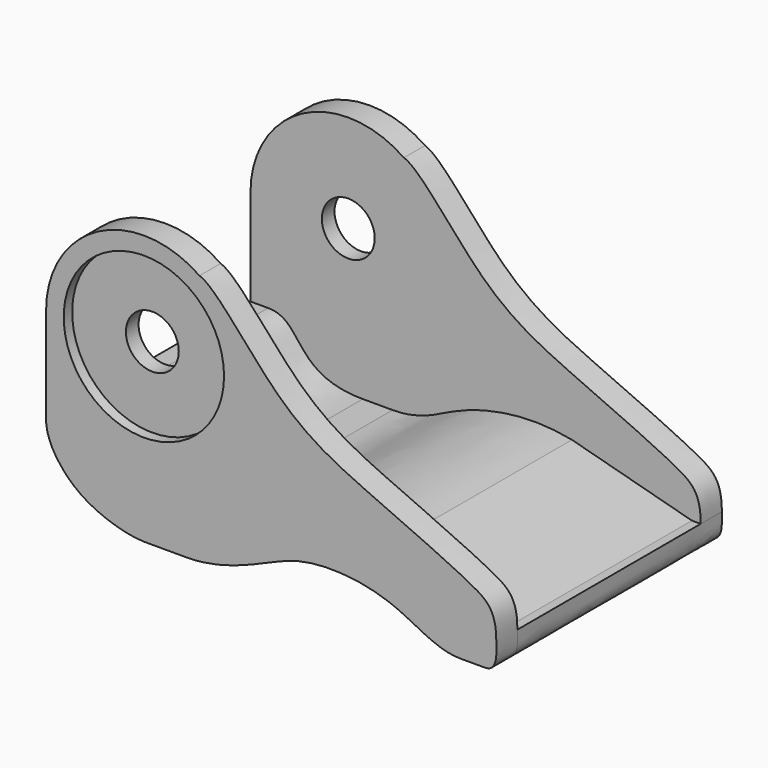
from build123d import *

# Parameters (mm, degrees)
F0_R     = 9.1
F0_R_2   = 3
F1_DEPTH = 3
F2_DEPTH = 32
F3_R     = 9.1
F3_R_2   = 3
F4_DEPTH = 3
F5_DEPTH = 1.2
F6_DEPTH = 1.2


# Not quite as in the source:
# - the dataset's text gives a spline's control points without its knots; the knots are read off the source's solid


with BuildPart() as f1:
    # F0 (on Front) → F1 (new body)
    with BuildSketch(Plane.XZ):
        with BuildLine():
            ThreePointArc((17.4131177763, 28.6298709707), (5.94566238, 29.330707182), (0, 19.5000000088))
            ThreePointArc((0, 19.5000000088), (11.0999999956, 8.4), (22.2, 19.5))
            ThreePointArc((22.2, 19.5), (20.93070718, 24.6543376239), (17.4131177763, 28.6298709707))
        make_face()
        with Locations((11.1, 19.5)):
            Circle(F0_R, mode=Mode.SUBTRACT)
        with BuildLine():
            Line((0, 19.5000000088), (0, 8.6))
            Line((0, 8.6), (2, 8.6))
            add(Edge.make_bspline(
                [(2, 8.6), (6.1005279422, 8.6), (4.7618634999, 3), (12.7434981987, 3)],
                knots=[0, 0, 0, 0, 12.1153932477, 12.1153932477, 12.1153932477, 12.1153932477], degree=3))
            Line((12.7434981987, 3), (16.1323161151, 3))
            add(Edge.make_bspline(
                [(36.4871002909, 6.6475654837), (33.250513749, 7.2772264404), (28.4821757642, 7.0333812875), (22.7707461668, 5.2870830071), (19.2182583484, 3), (16.1323161151, 3)],
                knots=[0, 0, 0, 0, 0.3619231415, 0.6598619876, 1, 1, 1, 1], degree=3))
            Line((36.4871002909, 6.6475654837), (50.1, 3))
            Line((50.1, 3), (51.1, 3))
            add(Edge.make_bspline(
                [(17.4131177763, 28.6298709707), (19.3173309809, 28.0148434267), (26.5141621262, 17.8054561903), (36.3055294732, 13.2861047363), (48.6152121195, 7.9013395134), (51.1, 6.0645417062), (51.1, 3)],
                knots=[0, 0, 0, 0, 0.2751149516, 0.5468245458, 0.818510602, 1, 1, 1, 1], degree=3))
            ThreePointArc((17.4131177763, 28.6298709707), (20.93070718, 24.6543376239), (22.2, 19.5))
            ThreePointArc((22.2, 19.5), (11.0999999956, 8.4), (0, 19.5000000088))
        make_face()
        with Locations((11.1, 19.5)):
            Circle(F0_R)
        with Locations((11.1, 19.5)):
            Circle(F0_R_2, mode=Mode.SUBTRACT)
        with BuildLine():
            add(Edge.make_bspline(
                [(36.4871002909, 6.6475654837), (33.250513749, 7.2772264404), (28.4821757642, 7.0333812875), (22.7707461668, 5.2870830071), (19.2182583484, 3), (16.1323161151, 3)],
                knots=[0, 0, 0, 0, 0.3619231415, 0.6598619876, 1, 1, 1, 1], degree=3))
            Line((16.1323161151, 3), (26.4085768866, 3))
            add(Edge.make_bspline(
                [(38.9945048839, 3), (37.6672047291, 3.494469873), (34.5451444696, 4.2269106386), (29.9007307702, 4.2671179583), (27.2729407986, 3.3486511872), (26.4085768866, 3)],
                knots=[0.2580240809, 0.2580240809, 0.2580240809, 0.2580240809, 0.396530844, 0.588257037, 0.6815213918, 0.6815213918, 0.6815213918, 0.6815213918], degree=3))
            Line((38.9945048839, 3), (50.1, 3))
            Line((50.1, 3), (36.4871002909, 6.6475654837))
        make_face()
        with BuildLine():
            Line((12.7434981987, 3), (3.1549932572, 3))
            add(Edge.make_bspline(
                [(11.1625680027, 0), (9.6983325574, 0), (6.2580804616, 0.8511709187), (3.8354236598, 2.4325332537), (3.1549932572, 3)],
                knots=[0, 0, 0, 0, 0.3599781606, 0.5310380634, 0.5310380634, 0.5310380634, 0.5310380634], degree=3))
            Line((11.1625680027, 0), (15.8881638199, 0))
            add(Edge.make_bspline(
                [(26.4085768866, 3), (25.5236936564, 2.6430721083), (22.55665667, 1.2844222732), (18.8493595825, 0), (15.8881638199, 0)],
                knots=[0.6815213918, 0.6815213918, 0.6815213918, 0.6815213918, 0.776999769, 1, 1, 1, 1], degree=3))
            Line((26.4085768866, 3), (16.1323161151, 3))
            Line((16.1323161151, 3), (12.7434981987, 3))
        make_face()
        with BuildLine():
            add(Edge.make_bspline(
                [(51.1, 3), (51.1, 1.8280865625), (51.3270497322, 0), (49.7638843954, 0)],
                knots=[0, 0, 0, 0, 3.2840835722, 3.2840835722, 3.2840835722, 3.2840835722], degree=3))
            Line((51.1, 3), (50.1, 3))
            Line((50.1, 3), (38.9945048839, 3))
            add(Edge.make_bspline(
                [(46.9955906657, 0), (44.6339409881, 0), (41.9557123636, 1.7760040782), (39.4711509433, 2.8224311844), (38.9945048839, 3)],
                knots=[0, 0, 0, 0, 0.2082849902, 0.2580240809, 0.2580240809, 0.2580240809, 0.2580240809], degree=3))
            Line((46.9955906657, 0), (49.7638843954, 0))
        make_face()
        with BuildLine():
            add(Edge.make_bspline(
                [(3.1549932572, 3), (2.7317734101, 3.3529577584), (2.3472268202, 3.728382037), (2, 4.1220149827)],
                knots=[0.5310380634, 0.5310380634, 0.5310380634, 0.5310380634, 0.6374353462, 0.6374353462, 0.6374353462, 0.6374353462], degree=3))
            Line((3.1549932572, 3), (12.7434981987, 3))
            add(Edge.make_bspline(
                [(2, 8.6), (6.1005279422, 8.6), (4.7618634999, 3), (12.7434981987, 3)],
                knots=[0, 0, 0, 0, 12.1153932477, 12.1153932477, 12.1153932477, 12.1153932477], degree=3))
            Line((2, 8.6), (2, 4.1220149827))
        make_face()
        with BuildLine():
            Line((2, 8.6), (0, 8.6))
            add(Edge.make_bspline(
                [(2, 4.1220149827), (1.7860800359, 4.3645248947), (0.6812014398, 5.7441151101), (0, 7.3046851351), (0, 8.6)],
                knots=[0.6374353462, 0.6374353462, 0.6374353462, 0.6374353462, 0.7029847265, 1, 1, 1, 1], degree=3))
            Line((2, 4.1220149827), (2, 8.6))
        make_face()
    extrude(amount=-F1_DEPTH)

    # F0 (on Front) → F2 (join)
    with BuildSketch(Plane.XZ):
        with BuildLine():
            Line((12.7434981987, 3), (3.1549932572, 3))
            add(Edge.make_bspline(
                [(11.1625680027, 0), (9.6983325574, 0), (6.2580804616, 0.8511709187), (3.8354236598, 2.4325332537), (3.1549932572, 3)],
                knots=[0, 0, 0, 0, 0.3599781606, 0.5310380634, 0.5310380634, 0.5310380634, 0.5310380634], degree=3))
            Line((11.1625680027, 0), (15.8881638199, 0))
            add(Edge.make_bspline(
                [(26.4085768866, 3), (25.5236936564, 2.6430721083), (22.55665667, 1.2844222732), (18.8493595825, 0), (15.8881638199, 0)],
                knots=[0.6815213918, 0.6815213918, 0.6815213918, 0.6815213918, 0.776999769, 1, 1, 1, 1], degree=3))
            Line((26.4085768866, 3), (16.1323161151, 3))
            Line((16.1323161151, 3), (12.7434981987, 3))
        make_face()
        with BuildLine():
            Line((2, 8.6), (0, 8.6))
            add(Edge.make_bspline(
                [(2, 4.1220149827), (1.7860800359, 4.3645248947), (0.6812014398, 5.7441151101), (0, 7.3046851351), (0, 8.6)],
                knots=[0.6374353462, 0.6374353462, 0.6374353462, 0.6374353462, 0.7029847265, 1, 1, 1, 1], degree=3))
            Line((2, 4.1220149827), (2, 8.6))
        make_face()
        with BuildLine():
            add(Edge.make_bspline(
                [(36.4871002909, 6.6475654837), (33.250513749, 7.2772264404), (28.4821757642, 7.0333812875), (22.7707461668, 5.2870830071), (19.2182583484, 3), (16.1323161151, 3)],
                knots=[0, 0, 0, 0, 0.3619231415, 0.6598619876, 1, 1, 1, 1], degree=3))
            Line((16.1323161151, 3), (26.4085768866, 3))
            add(Edge.make_bspline(
                [(38.9945048839, 3), (37.6672047291, 3.494469873), (34.5451444696, 4.2269106386), (29.9007307702, 4.2671179583), (27.2729407986, 3.3486511872), (26.4085768866, 3)],
                knots=[0.2580240809, 0.2580240809, 0.2580240809, 0.2580240809, 0.396530844, 0.588257037, 0.6815213918, 0.6815213918, 0.6815213918, 0.6815213918], degree=3))
            Line((38.9945048839, 3), (50.1, 3))
            Line((50.1, 3), (36.4871002909, 6.6475654837))
        make_face()
        with BuildLine():
            add(Edge.make_bspline(
                [(51.1, 3), (51.1, 1.8280865625), (51.3270497322, 0), (49.7638843954, 0)],
                knots=[0, 0, 0, 0, 3.2840835722, 3.2840835722, 3.2840835722, 3.2840835722], degree=3))
            Line((51.1, 3), (50.1, 3))
            Line((50.1, 3), (38.9945048839, 3))
            add(Edge.make_bspline(
                [(46.9955906657, 0), (44.6339409881, 0), (41.9557123636, 1.7760040782), (39.4711509433, 2.8224311844), (38.9945048839, 3)],
                knots=[0, 0, 0, 0, 0.2082849902, 0.2580240809, 0.2580240809, 0.2580240809, 0.2580240809], degree=3))
            Line((46.9955906657, 0), (49.7638843954, 0))
        make_face()
        with BuildLine():
            add(Edge.make_bspline(
                [(3.1549932572, 3), (2.7317734101, 3.3529577584), (2.3472268202, 3.728382037), (2, 4.1220149827)],
                knots=[0.5310380634, 0.5310380634, 0.5310380634, 0.5310380634, 0.6374353462, 0.6374353462, 0.6374353462, 0.6374353462], degree=3))
            Line((3.1549932572, 3), (12.7434981987, 3))
            add(Edge.make_bspline(
                [(2, 8.6), (6.1005279422, 8.6), (4.7618634999, 3), (12.7434981987, 3)],
                knots=[0, 0, 0, 0, 12.1153932477, 12.1153932477, 12.1153932477, 12.1153932477], degree=3))
            Line((2, 8.6), (2, 4.1220149827))
        make_face()
    extrude(amount=-F2_DEPTH)

    # F3 (on face) → F4 (join)
    with BuildSketch(Plane(origin=(0, 32, 0), x_dir=(-1, 0, 0), z_dir=(0, 1, 0))):
        with BuildLine():
            ThreePointArc((0, 19.5), (-5.9456623761, 29.33070718), (-17.4131177763, 28.6298709707))
            add(Edge.make_bspline(
                [(-17.4131177763, 28.6298709707), (-19.3173309809, 28.0148434267), (-26.5141621262, 17.8054561903), (-36.3055294732, 13.2861047363), (-48.6152121195, 7.9013395134), (-51.1, 6.0645417062), (-51.1, 3)],
                knots=[0, 0, 0, 0, 0.2751149516, 0.5468245458, 0.818510602, 1, 1, 1, 1], degree=3))
            Line((-51.1, 3), (-50.1, 3))
            Line((-50.1, 3), (-36.4871002909, 6.6475654837))
            add(Edge.make_bspline(
                [(-36.4871002909, 6.6475654837), (-33.250513749, 7.2772264404), (-28.4821757642, 7.0333812875), (-22.7707461668, 5.2870830071), (-19.2182583484, 3), (-16.1323161151, 3)],
                knots=[0, 0, 0, 0, 0.3619231415, 0.6598619876, 1, 1, 1, 1], degree=3))
            Line((-16.1323161151, 3), (-12.7434981987, 3))
            add(Edge.make_bspline(
                [(-2, 8.6), (-6.1005279422, 8.6), (-4.7618634999, 3), (-12.7434981987, 3)],
                knots=[0, 0, 0, 0, 12.1153932477, 12.1153932477, 12.1153932477, 12.1153932477], degree=3))
            Line((-2, 8.6), (0, 8.6))
            Line((0, 8.6), (0, 19.5))
        make_face()
        with Locations((-11.1, 19.5)):
            Circle(F3_R, mode=Mode.SUBTRACT)
        with Locations((-11.1, 19.5)):
            Circle(F3_R)
        with Locations((-11.1, 19.5)):
            Circle(F3_R_2, mode=Mode.SUBTRACT)
    extrude(amount=-F4_DEPTH)

    # F0 (on Front) → F5 (cut)
    with BuildSketch(Plane.XZ):
        with Locations((11.1, 19.5)):
            Circle(F0_R)
        with Locations((11.1, 19.5)):
            Circle(F0_R_2, mode=Mode.SUBTRACT)
    extrude(amount=-F5_DEPTH, mode=Mode.SUBTRACT)

    # F3 (on face) → F6 (cut)
    with BuildSketch(Plane(origin=(0, 32, 0), x_dir=(-1, 0, 0), z_dir=(0, 1, 0))):
        with Locations((-11.1, 19.5)):
            Circle(F3_R)
        with Locations((-11.1, 19.5)):
            Circle(F3_R_2, mode=Mode.SUBTRACT)
    extrude(amount=-F6_DEPTH, mode=Mode.SUBTRACT)


solid = f1.part
